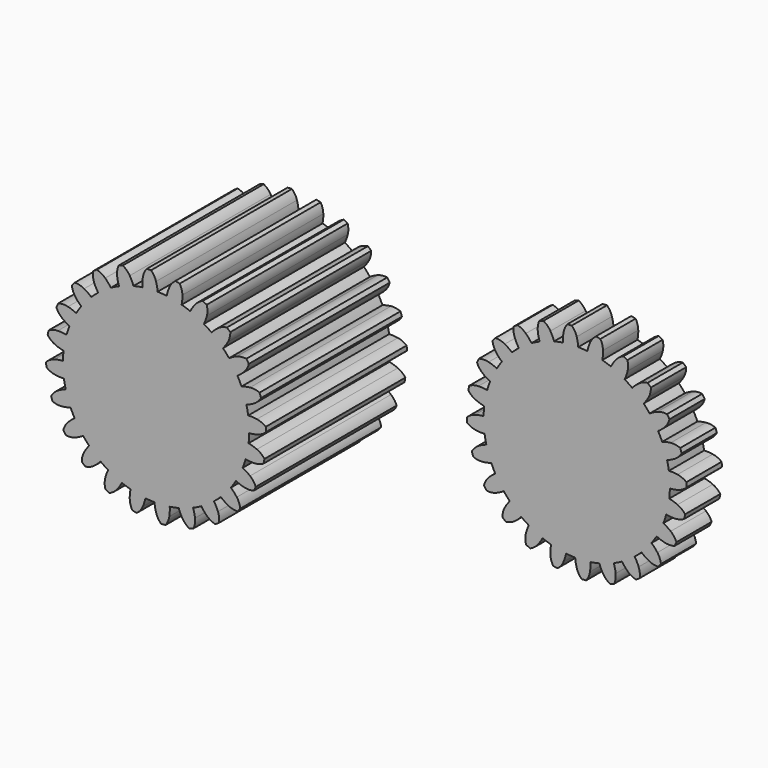
from build123d import *

# Parameters (mm, degrees)
F1_DEPTH        = 25.4
F1_COPIES_COUNT = 24
F4_DEPTH        = 101.6
F4_COPIES_COUNT = 24


# Not quite as in the source:
# - a feature of the source that left no trace in its solid (it failed there, or was rolled back) is left out
# - a pattern or mirror of a feature is missing from the dataset's text; its kind, count and spacing are read off the source's solid


with BuildPart() as f1:
    # F0 (on Front) → F1 (new body)
    with BuildSketch(Plane.XZ):
        with BuildLine():
            ThreePointArc((-7.8842675869, 53.139290225), (-35.0884247435, -40.6785974441), (53.721, 0))
            ThreePointArc((53.721, 0), (38.2966086664, 37.6738052983), (0.8807473744, 53.7137796572))
            ThreePointArc((0.8807473744, 53.7137796572), (-3.5135215054, 53.6059792153), (-7.8842675869, 53.139290225))
        make_face()
        with BuildLine():
            ThreePointArc((-7.8842675869, 53.139290225), (-3.5135215054, 53.6059792153), (0.8807473744, 53.7137796572))
            ThreePointArc((0.8807473744, 53.7137796572), (0.5824045109, 56.2191091266), (0, 58.674))
            ThreePointArc((0, 58.674), (-1.1288273681, 61.2344592008), (-2.8564405638, 63.4357213824))
            ThreePointArc((-2.8564405638, 63.4357213824), (-4.1529371344, 63.3615765173), (-5.448019844, 63.2658603022))
            ThreePointArc((-5.448019844, 63.2658603022), (-6.8735306986, 60.8579314517), (-7.6584938023, 58.1720357962))
            ThreePointArc((-7.6584938023, 58.1720357962), (-7.9154882038, 55.6621278115), (-7.8842675869, 53.139290225))
        make_face()
    extrude(amount=F1_DEPTH)

    # F1_copies: F1 ×24 about axis
    f1_copies_axis = Axis((0, 0, 0), (0, 1, 0))


with BuildPart() as f1_1:
    add(f1.part)
    for i in range(1, F1_COPIES_COUNT):
        add(f1.part.rotate(f1_copies_axis, i * 360 / F1_COPIES_COUNT))


with BuildPart() as f4:
    # F3 (on Front) → F4 (new body)
    with BuildSketch(Plane.XZ):
        with BuildLine():
            ThreePointArc((-189.5641571466, 53.139290225), (-216.7683143033, -40.6785974441), (-127.9588895597, 0))
            ThreePointArc((-127.9588895597, 0), (-143.3832808933, 37.6738052983), (-180.7991421854, 53.7137796572))
            ThreePointArc((-180.7991421854, 53.7137796572), (-185.1934110651, 53.6059792153), (-189.5641571466, 53.139290225))
        make_face()
        with BuildLine():
            ThreePointArc((-189.5641571466, 53.139290225), (-185.1934110651, 53.6059792153), (-180.7991421854, 53.7137796572))
            ThreePointArc((-180.7991421854, 53.7137796572), (-181.0974850489, 56.2191091266), (-181.6798895597, 58.674))
            ThreePointArc((-181.6798895597, 58.674), (-182.8087169279, 61.2344592008), (-184.5363301236, 63.4357213824))
            ThreePointArc((-184.5363301236, 63.4357213824), (-185.8325446972, 63.3572740763), (-187.1279094037, 63.2658603022))
            ThreePointArc((-187.1279094037, 63.2658603022), (-188.5534202584, 60.8579314517), (-189.3383833621, 58.1720357962))
            ThreePointArc((-189.3383833621, 58.1720357962), (-189.5953777636, 55.6621278115), (-189.5641571466, 53.139290225))
        make_face()
    extrude(amount=F4_DEPTH)

    # F4_copies: F4 ×24 about axis
    f4_copies_axis = Axis((-181.679889, 0, -1e-06), (0, 1, 0))


with BuildPart() as f4_1:
    add(f4.part)
    for i in range(1, F4_COPIES_COUNT):
        add(f4.part.rotate(f4_copies_axis, i * 360 / F4_COPIES_COUNT))


solid = Compound([f1_1.part, f4_1.part])
